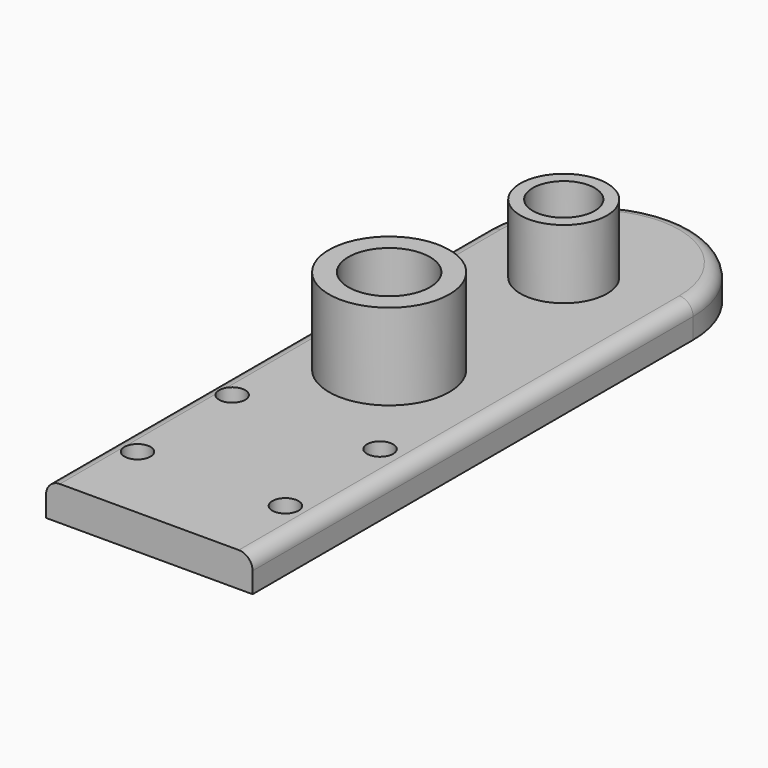
from build123d import *

# Parameters (mm, degrees)
F1_DEPTH     = 12.7
F2_R         = 4.826
F3_DEPTH     = 12.701
F4_R         = 22.225
F5_DEPTH     = 31.75
F6_R         = 16.002
F6_R_2       = 11.4285628251
F7_DEPTH     = 25.4
F8_R         = 15.0651318588
F9_DEPTH     = 31.75
F10_T1_DEPTH = 215.9
F10_T4_ANGLE = 180


# Not quite as in the source:
# - a fillet or chamfer that OpenCascade refuses, or shapes differently, is made with other operations: its cross-section is extruded or revolved along the edge and cut away or added


with BuildPart() as f1:
    # F0 (on Top) → F1 (new body)
    with BuildSketch(Plane.XY):
        with BuildLine():
            Line((-28.8097388059, 45.6853893078), (-28.8097388059, -157.5146106922))
            Line((-28.8097388059, -157.5146106922), (47.3902611941, -157.5146106922))
            Line((47.3902611941, -157.5146106922), (47.3902611941, 45.6853893078))
            ThreePointArc((47.3902611941, 45.6853893078), (9.2902611941, 83.7853893078), (-28.8097388059, 45.6853893078))
        make_face()
    extrude(amount=F1_DEPTH)

    # F2 (on face) → F3 (cut, through all)
    with BuildSketch(Plane.XY.offset(12.7)):
        with Locations((-18.8133654982, -127.8345082872)):
            Circle(F2_R)
        with Locations((35.5419658125, -127.5648898334)):
            Circle(F2_R)
        with Locations((-19.6402604571, -83.1381565264)):
            Circle(F2_R)
        with Locations((34.7150708535, -82.8685380725)):
            Circle(F2_R)
    extrude(amount=-F3_DEPTH, mode=Mode.SUBTRACT)

    # F4 (on face) → F5 (join)
    with BuildSketch(Plane.XY.offset(12.7)):
        with Locations((5.8846990578, -42.6385067403)):
            Circle(F4_R)
    extrude(amount=F5_DEPTH)

    # F6 (on face) → F7 (join)
    with BuildSketch(Plane.XY.offset(12.7)):
        with Locations((9.203276597, 33.7460897863)):
            Circle(F6_R)
        with Locations((9.203276597, 33.7460897863)):
            Circle(F6_R_2, mode=Mode.SUBTRACT)
    extrude(amount=F7_DEPTH)

    # F8 (on face) → F9 (cut)
    with BuildSketch(Plane.XY.offset(44.45)):
        with Locations((5.8846990578, -42.6385067403)):
            Circle(F8_R)
    extrude(amount=-F9_DEPTH, mode=Mode.SUBTRACT)

    # F10: fillet of radius 5.08 on 3 edges, made by hand

    # F10_s2 → F10_t1 (cut)
    with BuildSketch(Plane.XZ.offset(-45.6853893078)):
        with BuildLine():
            ThreePointArc((42.3102611941, 12.7), (45.9023636425, 11.2121024484), (47.3902611941, 7.62))
            Line((47.3902611941, 7.62), (47.3902611941, 12.7))
            Line((47.3902611941, 12.7), (42.3102611941, 12.7))
        make_face()
        with BuildLine():
            ThreePointArc((-28.8097388059, 7.62), (-27.3218412543, 11.2121024484), (-23.7297388059, 12.7))
            Line((-23.7297388059, 12.7), (-28.8097388059, 12.7))
            Line((-28.8097388059, 12.7), (-28.8097388059, 7.62))
        make_face()
    extrude(amount=F10_T1_DEPTH, mode=Mode.SUBTRACT)

    # F10_s3 → F10_t4 (revolve, cut)
    with BuildSketch(Plane.XZ.offset(-45.6853893078)):
        with BuildLine():
            ThreePointArc((47.3902611941, 7.62), (45.9023636425, 11.2121024484), (42.3102611941, 12.7))
            Line((42.3102611941, 12.7), (47.3902611941, 12.7))
            Line((47.3902611941, 12.7), (47.3902611941, 7.62))
        make_face()
    revolve(axis=Axis((9.2902611941, 45.6853893078, 12.7), (0, 0, 1)), revolution_arc=F10_T4_ANGLE, mode=Mode.SUBTRACT)


solid = f1.part
